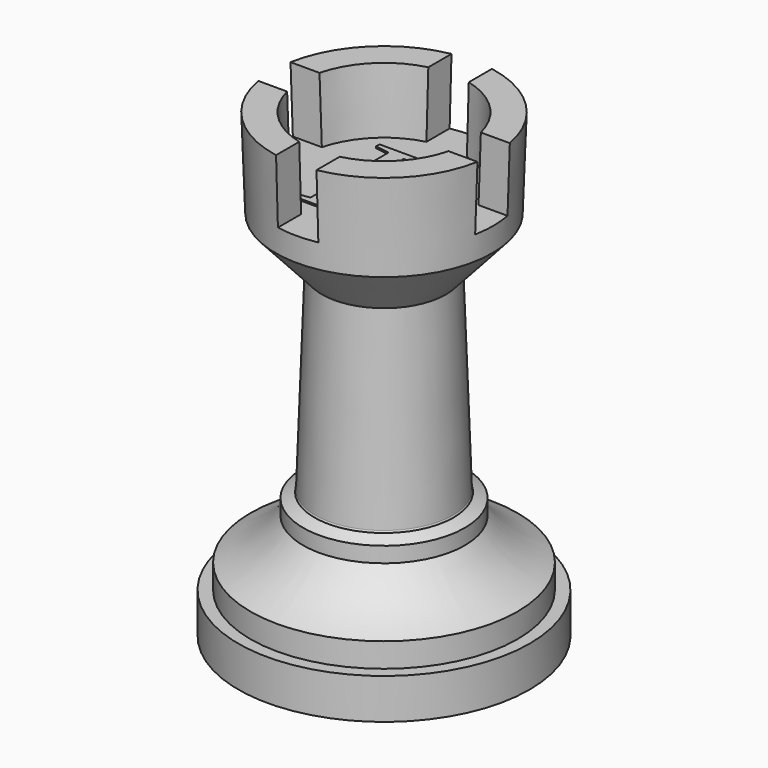
from build123d import *

# Parameters (mm, degrees)
F2_W         = 15.6068325573
F2_H         = 5
F2_W_2       = 5
F2_H_2       = 15.8233622873
F2_W_3       = 16.7265002215
F2_H_3       = 16.0099732542
F3_DEPTH     = 7.9961266162
F4_TEXT_SIZE = 20.8333333333
F5_DEPTH     = 0.2
F6_TEXT_SIZE = 35.2777777778
F7_DEPTH     = 0.4


# Not quite as in the source:
# - Text() gives the source's letters only with a copy of the font that has no kerning and outlines rounded to 1/6400 em; it was checked with that copy


with BuildPart() as f1:
    # F0 (on Front) → F1 (revolve)
    with BuildSketch(Plane.XZ):
        with BuildLine():
            Line((18, 0), (16.5, 0))
            Line((16.5, 0), (16.5, 3))
            ThreePointArc((16.5, 3), (12.8660278936, 5.0560559388), (10, 8.0923371193))
            Line((10, 8.0923371193), (10, 10))
            Line((10, 10), (8.5917271114, 10.6566884327))
            ThreePointArc((8.5917271114, 10.6566884327), (8.5453800175, 10.7684182859), (8.5, 10.8805444079))
            Line((8.5, 10.8805444079), (7.670398013, 34.6372370304))
            Line((7.670398013, 34.6372370304), (13.3950675092, 40.9951266162))
            Line((13.3950675092, 40.9951266162), (13.7791959736, 51.9951266162))
            Line((13.7791959736, 51.9951266162), (10.2791959736, 51.9951266162))
            Line((10.2791959736, 51.9951266162), (10, 44))
            Line((10, 44), (0, 44))
            Line((0, 44), (0, 0))
            Line((0, 0), (0, -5))
            Line((0, -5), (18, -5))
            Line((18, -5), (18, 0))
        make_face()
    revolve(axis=Axis((0, 0, 22), (0, 0, -1)))

    # F2 (on face) → F3 (cut, through all)
    with BuildSketch(Plane.XY.offset(44)):
        with Locations((-10.3034162787, 0)):
            Rectangle(F2_W, F2_H)
        with Locations((0, 10.4116811437)):
            Rectangle(F2_W_2, F2_H_2)
        Rectangle(F2_W_2, F2_H)
        with Locations((10.8632501107, 0)):
            Rectangle(F2_W_3, F2_H)
        with Locations((0, -10.5049866271)):
            Rectangle(F2_W_2, F2_H_3)
    extrude(amount=F3_DEPTH, mode=Mode.SUBTRACT)

    # F4 (on face) → F5 (join)
    with BuildSketch(Plane.XY.offset(44)):
        with Locations((-6.0677083333, -7.5)):
            Text('F', F4_TEXT_SIZE, font='Tinos', text_align=(TextAlign.LEFT, TextAlign.BOTTOM))
    extrude(amount=F5_DEPTH)

    # F6 (on face) → F7 (cut)
    with BuildSketch(Plane(origin=(0, 0, -5), x_dir=(1, 0, 0), z_dir=(0, 0, -1))):
        with Locations((-12.6421223958, -12.7)):
            Text('∞', F6_TEXT_SIZE, font='Open Sans', font_style=FontStyle.BOLD, text_align=(TextAlign.LEFT, TextAlign.BOTTOM))
    extrude(amount=-F7_DEPTH, mode=Mode.SUBTRACT)


solid = f1.part
